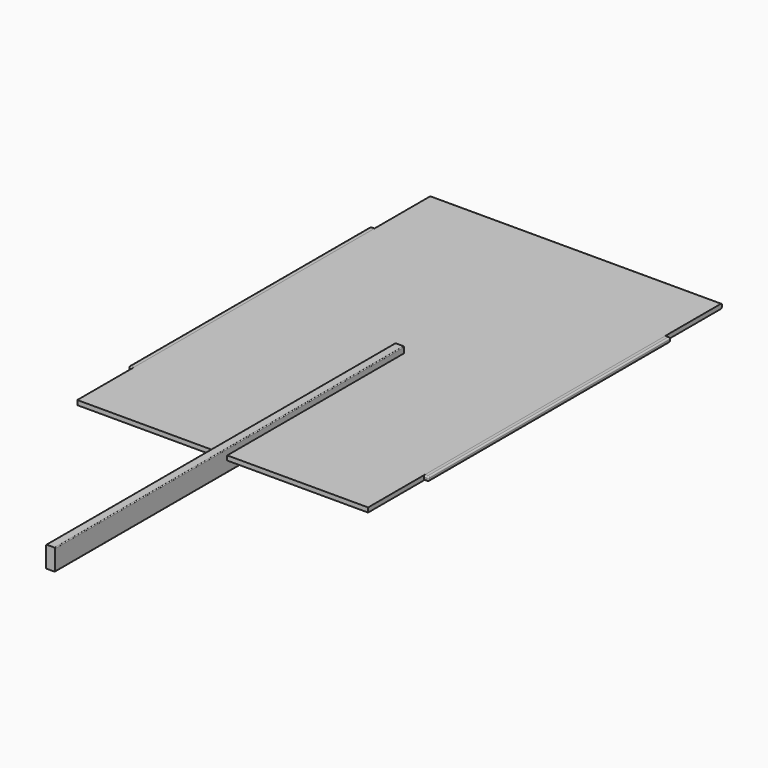
from build123d import *

# Parameters (mm, degrees)
F1_DEPTH     = 1219.2
F2_DEPTH     = 1143
F3_W         = 1257.3
F3_H         = 1270
F4_DEPTH     = 19.05
F5_R         = 6.35
F6_T1_DEPTH  = 1244.6
F6_T3_DEPTH  = 6.35
F6_S7_W      = 6.477
F6_S7_H      = 6.477
F6_T8_DEPTH  = 6.477
F6_S13_W     = 6.477
F6_S13_H     = 6.477
F6_T14_DEPTH = 6.477
F6_S19_W     = 6.477
F6_S19_H     = 6.477
F6_T20_DEPTH = 6.477
F6_S25_W     = 6.477
F6_S25_H     = 6.477
F6_T26_DEPTH = 6.477
F6_T30_ANGLE = 90
F6_T32_ANGLE = 90
F6_T34_ANGLE = 90
F6_T36_ANGLE = 90
F7_DEPTH     = 1828.8
F8_W         = 1219.2
F8_H         = 1854.2
F9_DEPTH     = 19.05
F10_R        = 6.35


# Not quite as in the source:
# - a fillet or chamfer that OpenCascade refuses, or shapes differently, is made with other operations: its cross-section is extruded or revolved along the edge and cut away or added


with BuildPart() as f1:
    # F0 (on Front) → F1 (new body)
    with BuildSketch(Plane.XZ):
        with BuildLine():
            ThreePointArc((19.05, 41.275), (18.1200640303, 43.5200640303), (15.875, 44.45))
            Line((15.875, 44.45), (-15.875, 44.45))
            ThreePointArc((-15.875, 44.45), (-18.1200640303, 43.5200640303), (-19.05, 41.275))
            Line((-19.05, 41.275), (-19.05, -41.275))
            ThreePointArc((-19.05, -41.275), (-18.1200640303, -43.5200640303), (-15.875, -44.45))
            Line((-15.875, -44.45), (15.875, -44.45))
            ThreePointArc((15.875, -44.45), (18.1200640303, -43.5200640303), (19.05, -41.275))
            Line((19.05, -41.275), (19.05, 41.275))
        make_face()
    extrude(amount=F1_DEPTH)


with BuildPart() as f2:
    # F0 (on Front) → F2 (new body)
    with BuildSketch(Plane.XZ):
        with BuildLine():
            ThreePointArc((19.05, 41.275), (18.1200640303, 43.5200640303), (15.875, 44.45))
            Line((15.875, 44.45), (-15.875, 44.45))
            ThreePointArc((-15.875, 44.45), (-18.1200640303, 43.5200640303), (-19.05, 41.275))
            Line((-19.05, 41.275), (-19.05, -41.275))
            ThreePointArc((-19.05, -41.275), (-18.1200640303, -43.5200640303), (-15.875, -44.45))
            Line((-15.875, -44.45), (15.875, -44.45))
            ThreePointArc((15.875, -44.45), (18.1200640303, -43.5200640303), (19.05, -41.275))
            Line((19.05, -41.275), (19.05, 41.275))
        make_face()
    extrude(amount=F2_DEPTH)


with BuildPart() as f4:
    # F3 (on Top) → F4 (new body)
    with BuildSketch(Plane.XY):
        Rectangle(F3_W, F3_H)
    extrude(amount=F4_DEPTH)

    # F5
    f5_edges = [f4.edges().sort_by_distance(p)[0] for p in [
        (-628.65, 0, 19.05),
        (0, -635, 19.05),
        (0, 635, 19.05),
        (628.65, 0, 19.05),
        (628.65, 0, 0),
        (-628.65, 0, 0),
    ]]
    fillet(f5_edges, radius=F5_R)

    # F6: fillet of radius 6.35 on 2 edges, made by hand

    # F6_s2 → F6_t1 (cut)
    with BuildSketch(Plane.YZ.offset(-622.3)):
        with BuildLine():
            ThreePointArc((-628.65, 0), (-633.1401280605, 1.8598719395), (-635, 6.35))
            Line((-635, 6.35), (-635.127, 6.35))
            Line((-635.127, 6.35), (-635.127, -0.127))
            Line((-635.127, -0.127), (-628.65, -0.127))
            Line((-628.65, -0.127), (-628.65, 0))
        make_face()
        with BuildLine():
            ThreePointArc((635, 6.35), (633.1401280605, 1.8598719395), (628.65, 0))
            Line((628.65, 0), (628.65, -0.127))
            Line((628.65, -0.127), (635.127, -0.127))
            Line((635.127, -0.127), (635.127, 6.35))
            Line((635.127, 6.35), (635, 6.35))
        make_face()
    extrude(amount=F6_T1_DEPTH, mode=Mode.SUBTRACT)

    # F6_s4 → F6_t3 (cut)
    with BuildSketch(Plane.XY.offset(6.35)):
        with BuildLine():
            ThreePointArc((-622.3, 635), (-626.7901280605, 633.1401280605), (-628.65, 628.65))
            Line((-628.65, 628.65), (-628.777, 628.65))
            Line((-628.777, 628.65), (-628.777, 635.127))
            Line((-628.777, 635.127), (-622.3, 635.127))
            Line((-622.3, 635.127), (-622.3, 635))
        make_face()
        with BuildLine():
            ThreePointArc((622.3, 635), (626.7901280605, 633.1401280605), (628.65, 628.65))
            Line((628.65, 628.65), (628.777, 628.65))
            Line((628.777, 628.65), (628.777, 635.127))
            Line((628.777, 635.127), (622.3, 635.127))
            Line((622.3, 635.127), (622.3, 635))
        make_face()
        with BuildLine():
            ThreePointArc((628.65, -628.65), (626.7901280605, -633.1401280605), (622.3, -635))
            Line((622.3, -635), (622.3, -635.127))
            Line((622.3, -635.127), (628.777, -635.127))
            Line((628.777, -635.127), (628.777, -628.65))
            Line((628.777, -628.65), (628.65, -628.65))
        make_face()
        with BuildLine():
            ThreePointArc((-628.65, -628.65), (-626.7901280605, -633.1401280605), (-622.3, -635))
            Line((-622.3, -635), (-622.3, -635.127))
            Line((-622.3, -635.127), (-628.777, -635.127))
            Line((-628.777, -635.127), (-628.777, -628.65))
            Line((-628.777, -628.65), (-628.65, -628.65))
        make_face()
    extrude(amount=F6_T3_DEPTH, mode=Mode.SUBTRACT)


with BuildPart() as f6_tool6:
    # F6_s7 → F6_t8 (new body)
    with BuildSketch(Plane.XZ.offset(-628.65)):
        with Locations((-625.5385, 15.9385)):
            Rectangle(F6_S7_W, F6_S7_H)
    extrude(amount=-F6_T8_DEPTH)

    # F6_s9 → F6_t10 (revolve, cut)
    with BuildSketch(Plane(origin=(-622.3, 628.65, 12.7), x_dir=(0.7071067812, 0, -0.7071067812), z_dir=(0.7071067812, 0, 0.7071067812))):
        with BuildLine():
            ThreePointArc((0, -6.35), (6.35, 0), (0, 6.35))
            Line((0, 6.35), (0, -6.35))
        make_face()
    revolve(axis=Axis((-622.3, 628.65, 12.7), (0, 1, 0)), mode=Mode.SUBTRACT)


with BuildPart() as f4_1:
    add(f4.part)

    # F6_t5: cut F6_tool6
    add(f6_tool6.part, mode=Mode.SUBTRACT)


with BuildPart() as f6_tool12:
    # F6_s13 → F6_t14 (new body)
    with BuildSketch(Plane.XZ.offset(-628.65)):
        with Locations((625.5385, 15.9385)):
            Rectangle(F6_S13_W, F6_S13_H)
    extrude(amount=-F6_T14_DEPTH)

    # F6_s15 → F6_t16 (revolve, cut)
    with BuildSketch(Plane(origin=(622.3, 628.65, 12.7), x_dir=(-0.7071067812, 0, -0.7071067812), z_dir=(0.7071067812, 0, -0.7071067812))):
        with BuildLine():
            ThreePointArc((0, -6.35), (6.35, 0), (0, 6.35))
            Line((0, 6.35), (0, -6.35))
        make_face()
    revolve(axis=Axis((622.3, 628.65, 12.7), (0, 1, 0)), mode=Mode.SUBTRACT)


with BuildPart() as f4_2:
    add(f4_1.part)

    # F6_t11: cut F6_tool12
    add(f6_tool12.part, mode=Mode.SUBTRACT)


with BuildPart() as f6_tool18:
    # F6_s19 → F6_t20 (new body)
    with BuildSketch(Plane.YZ.offset(622.3)):
        with Locations((-631.8885, 15.9385)):
            Rectangle(F6_S19_W, F6_S19_H)
    extrude(amount=F6_T20_DEPTH)

    # F6_s21 → F6_t22 (revolve, cut)
    with BuildSketch(Plane(origin=(622.3, -628.65, 12.7), x_dir=(0, 0.7071067812, -0.7071067812), z_dir=(0, -0.7071067812, -0.7071067812))):
        with BuildLine():
            ThreePointArc((0, -6.35), (6.35, 0), (0, 6.35))
            Line((0, 6.35), (0, -6.35))
        make_face()
    revolve(axis=Axis((622.3, -628.65, 12.7), (1, 0, 0)), mode=Mode.SUBTRACT)


with BuildPart() as f4_3:
    add(f4_2.part)

    # F6_t17: cut F6_tool18
    add(f6_tool18.part, mode=Mode.SUBTRACT)


with BuildPart() as f6_tool24:
    # F6_s25 → F6_t26 (new body)
    with BuildSketch(Plane.YZ.offset(-622.3)):
        with Locations((-631.8885, 15.9385)):
            Rectangle(F6_S25_W, F6_S25_H)
    extrude(amount=-F6_T26_DEPTH)

    # F6_s27 → F6_t28 (revolve, cut)
    with BuildSketch(Plane(origin=(-622.3, -628.65, 12.7), x_dir=(0, 0.7071067812, -0.7071067812), z_dir=(0, 0.7071067812, 0.7071067812))):
        with BuildLine():
            ThreePointArc((0, -6.35), (6.35, 0), (0, 6.35))
            Line((0, 6.35), (0, -6.35))
        make_face()
    revolve(axis=Axis((-622.3, -628.65, 12.7), (-1, 0, 0)), mode=Mode.SUBTRACT)


with BuildPart() as f4_4:
    add(f4_3.part)

    # F6_t23: cut F6_tool24
    add(f6_tool24.part, mode=Mode.SUBTRACT)

    # F6_s29 → F6_t30 (revolve, cut)
    with BuildSketch(Plane.XY.offset(6.35)):
        with BuildLine():
            ThreePointArc((622.3, 635), (626.7901280605, 633.1401280605), (628.65, 628.65))
            Line((628.65, 628.65), (628.777, 628.65))
            Line((628.777, 628.65), (628.777, 635.127))
            Line((628.777, 635.127), (622.3, 635.127))
            Line((622.3, 635.127), (622.3, 635))
        make_face()
    revolve(axis=Axis((622.3, 635, 6.35), (0, 1, 0)), revolution_arc=F6_T30_ANGLE, mode=Mode.SUBTRACT)

    # F6_s31 → F6_t32 (revolve, cut)
    with BuildSketch(Plane.XY.offset(6.35)):
        with BuildLine():
            ThreePointArc((-622.3, 635), (-626.7901280605, 633.1401280605), (-628.65, 628.65))
            Line((-628.65, 628.65), (-628.777, 628.65))
            Line((-628.777, 628.65), (-628.777, 635.127))
            Line((-628.777, 635.127), (-622.3, 635.127))
            Line((-622.3, 635.127), (-622.3, 635))
        make_face()
    revolve(axis=Axis((-622.3, 635, 6.35), (0, -1, 0)), revolution_arc=F6_T32_ANGLE, mode=Mode.SUBTRACT)

    # F6_s33 → F6_t34 (revolve, cut)
    with BuildSketch(Plane.XY.offset(6.35)):
        with BuildLine():
            ThreePointArc((-628.65, -628.65), (-626.7901280605, -633.1401280605), (-622.3, -635))
            Line((-622.3, -635), (-622.3, -635.127))
            Line((-622.3, -635.127), (-628.777, -635.127))
            Line((-628.777, -635.127), (-628.777, -628.65))
            Line((-628.777, -628.65), (-628.65, -628.65))
        make_face()
    revolve(axis=Axis((-622.3, -635, 6.35), (0, -1, 0)), revolution_arc=F6_T34_ANGLE, mode=Mode.SUBTRACT)

    # F6_s35 → F6_t36 (revolve, cut)
    with BuildSketch(Plane.XY.offset(6.35)):
        with BuildLine():
            ThreePointArc((628.65, -628.65), (626.7901280605, -633.1401280605), (622.3, -635))
            Line((622.3, -635), (622.3, -635.127))
            Line((622.3, -635.127), (628.777, -635.127))
            Line((628.777, -635.127), (628.777, -628.65))
            Line((628.777, -628.65), (628.65, -628.65))
        make_face()
    revolve(axis=Axis((622.3, -635, 6.35), (0, 1, 0)), revolution_arc=F6_T36_ANGLE, mode=Mode.SUBTRACT)


with BuildPart() as f7:
    # F0 (on Front) → F7 (new body)
    with BuildSketch(Plane.XZ):
        with BuildLine():
            ThreePointArc((19.05, 41.275), (18.1200640303, 43.5200640303), (15.875, 44.45))
            Line((15.875, 44.45), (-15.875, 44.45))
            ThreePointArc((-15.875, 44.45), (-18.1200640303, 43.5200640303), (-19.05, 41.275))
            Line((-19.05, 41.275), (-19.05, -41.275))
            ThreePointArc((-19.05, -41.275), (-18.1200640303, -43.5200640303), (-15.875, -44.45))
            Line((-15.875, -44.45), (15.875, -44.45))
            ThreePointArc((15.875, -44.45), (18.1200640303, -43.5200640303), (19.05, -41.275))
            Line((19.05, -41.275), (19.05, 41.275))
        make_face()
    extrude(amount=F7_DEPTH)


with BuildPart() as f9:
    # F8 (on Top) → F9 (new body)
    with BuildSketch(Plane.XY):
        Rectangle(F8_W, F8_H)
    extrude(amount=F9_DEPTH)

    # F10
    f10_edges = [f9.edges().sort_by_distance(p)[0] for p in [
        (0, 927.1, 19.05),
        (0, 927.1, 0),
    ]]
    fillet(f10_edges, radius=F10_R)


solid = Compound([f1.part, f2.part, f4_4.part, f7.part, f9.part])
